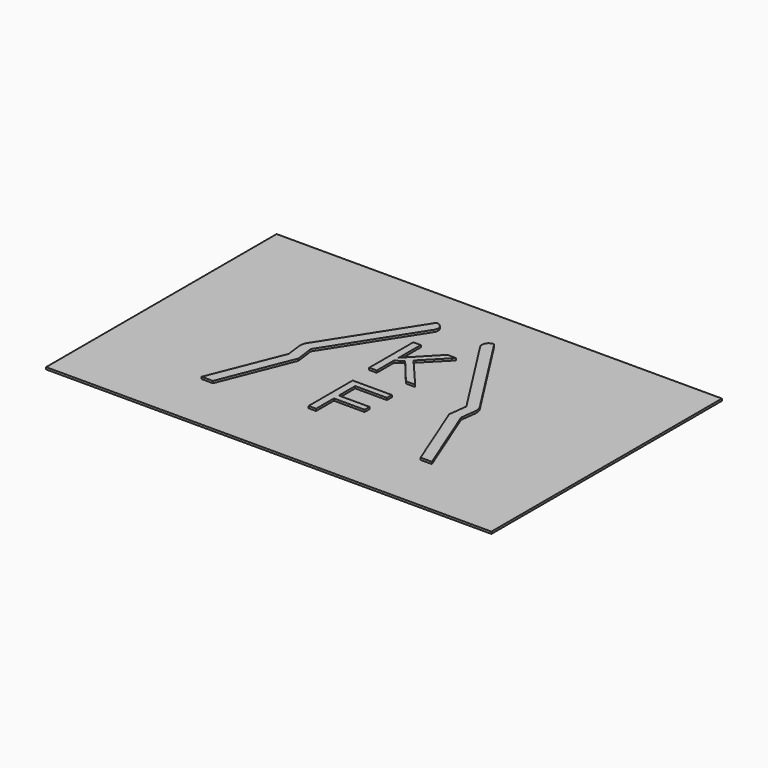
from build123d import *

# Parameters (mm, degrees)
F0_W         = 85
F0_H         = 55
F1_DEPTH     = 0.4
F2_TEXT_SIZE = 15.2777777778
F3_DEPTH     = 0.4


# Not quite as in the source:
# - Text() gives the source's letters only with a copy of the font that has no kerning and outlines rounded to 1/6400 em; it was checked with that copy


with BuildPart() as f1:
    # F0 (on Top) → F1 (new body)
    with BuildSketch(Plane.XY):
        Rectangle(F0_W, F0_H)
    extrude(amount=F1_DEPTH)

    # F2 (on face) → F3 (join)
    with BuildSketch(Plane.XY.offset(0.4)):
        with BuildLine():
            ThreePointArc((-4.3852040848, 17.4577778213), (-4.3627646639, 18.7727850902), (-5.5268212256, 19.3849288363))
            Line((-5.5268212256, 19.3849288363), (-16.4571341718, 2.2917793607))
            ThreePointArc((-16.4571341718, 2.2917793607), (-16.7723678199, 1.5365343487), (-16.8119416656, 0.7190986071))
            Line((-16.8119416656, 0.7190986071), (-16.4468014641, -2.1834347388))
            Line((-16.4468014641, -2.1834347388), (-21.9669759133, -16.0401687026))
            Line((-21.9669759133, -16.0401687026), (-19.8141149992, -16.0401687026))
            Line((-19.8141149992, -16.0401687026), (-14.3981348838, -2.4449832055))
            Line((-14.3981348838, -2.4449832055), (-14.8275820384, 0.9687320782))
            ThreePointArc((-14.8275820384, 0.9687320782), (-14.8214021692, 1.0963832045), (-14.7721751435, 1.2143225991))
            Line((-14.7721751435, 1.2143225991), (-4.3852040848, 17.4577778213))
        make_face()
        with BuildLine():
            Line((4.3852040848, 17.4577778213), (14.7721751435, 1.2143225991))
            ThreePointArc((14.7721751435, 1.2143225991), (14.8214021692, 1.0963832045), (14.8275820384, 0.9687320782))
            Line((14.8275820384, 0.9687320782), (14.3981348838, -2.4449832055))
            Line((14.3981348838, -2.4449832055), (19.8141149992, -16.0401687026))
            Line((19.8141149992, -16.0401687026), (21.9669759133, -16.0401687026))
            Line((21.9669759133, -16.0401687026), (16.4468014641, -2.1834347388))
            Line((16.4468014641, -2.1834347388), (16.8119416656, 0.7190986071))
            ThreePointArc((16.8119416656, 0.7190986071), (16.7723678199, 1.5365343487), (16.4571341718, 2.2917793607))
            Line((16.4571341718, 2.2917793607), (5.5268212256, 19.3849288363))
            ThreePointArc((5.5268212256, 19.3849288363), (4.3627646639, 18.7727850902), (4.3852040848, 17.4577778213))
        make_face()
        with Locations((-5.5393880208, 1.8367207944)):
            Text('K', F2_TEXT_SIZE, font='Arimo', text_align=(TextAlign.LEFT, TextAlign.BOTTOM))
        with Locations((-4.8900824653, -13.4449832055)):
            Text('F', F2_TEXT_SIZE, font='Arimo', text_align=(TextAlign.LEFT, TextAlign.BOTTOM))
    extrude(amount=F3_DEPTH)


solid = f1.part
